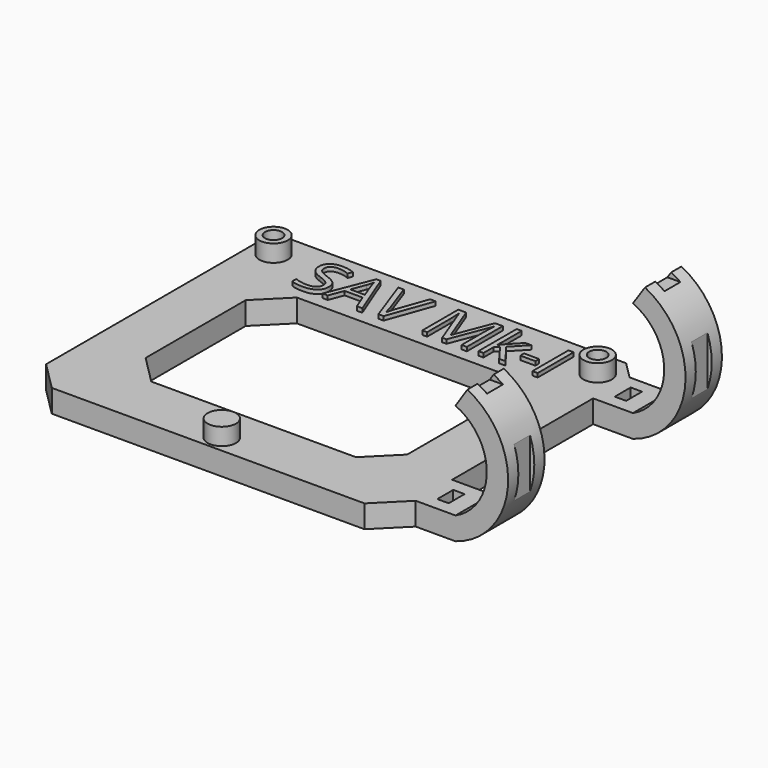
from build123d import *

# Parameters (mm, degrees)
F0_W          = 65
F0_H          = 55
F1_DEPTH      = 4
F2_W          = 46
F2_H          = 32
F3_DEPTH      = 4
F4_SIZE       = 5
F5_R          = 2.5
F6_DEPTH      = 3
F9_D          = 3
F9_ON_F8_D    = 3
F10_W         = 7
F10_H         = 8
F11_DEPTH     = 4
F12_SIZE      = 4.99999
F13_SIZE      = 2.99999
F14_SIZE      = 5
F15_SIZE      = 3
F16_TEXT_SIZE = 11.0753294494
F17_DEPTH     = 0.7
F19_DEPTH     = 8
F21_DEPTH     = 8
F22_W         = 7.0721879601
F22_H         = 3.5
F22_W_2       = 5.6506387591
F23_DEPTH     = 24.1616448952
F24_W         = 2
F24_H         = 3.5
F25_DEPTH     = 4.001
F26_W         = 3.5
F26_H         = 5.8661212551
F26_H_2       = 5.611290465
F27_DEPTH     = 81.2529563753


# Not quite as in the source:
# - a fillet or chamfer is up to 0.001 mm smaller than in the source, because OpenCascade refuses the exact size
# - Text() gives the source's letters only with a copy of the font that has no kerning and outlines rounded to 1/6400 em; it was checked with that copy


with BuildPart() as f1:
    # F0 (on Top) → F1 (new body)
    with BuildSketch(Plane.XY):
        with Locations((32.5, 27.5)):
            Rectangle(F0_W, F0_H)
    extrude(amount=F1_DEPTH)

    # F2 (on face) → F3 (cut, through all)
    with BuildSketch(Plane.XY.offset(4)):
        with Locations((32.5, 26)):
            Rectangle(F2_W, F2_H)
    extrude(amount=-F3_DEPTH, mode=Mode.SUBTRACT)

    # F4
    f4_edges = [f1.edges().sort_by_distance(p)[0] for p in [
        (9.5, 42, 2),
        (55.5, 42, 2),
        (9.5, 10, 2),
        (55.5, 10, 2),
    ]]
    chamfer(f4_edges, length=F4_SIZE)

    # F5 (on face) → F6 (join)
    with BuildSketch(Plane.XY.offset(4)):
        with Locations((32.5, 3)):
            Circle(F5_R)
        with Locations((4, 50)):
            Circle(F5_R)
        with Locations((61, 50)):
            Circle(F5_R)
    extrude(amount=F6_DEPTH)

    # F9 (through all)
    with Locations(Plane.XY.offset(7)):
        with Locations((4, 50)):
            Hole(F9_D / 2)

    # F9 on F8 (through all)
    with Locations(Plane.XY.offset(7)):
        with Locations((61, 50)):
            Hole(F9_ON_F8_D / 2)

    # F10 (on face) → F11 (join)
    with BuildSketch(Plane.XY.offset(4)):
        with Locations((68.5, 48)):
            Rectangle(F10_W, F10_H)
        with Locations((68.5, 9)):
            Rectangle(F10_W, F10_H)
    extrude(amount=-F11_DEPTH)

    # F12 (size 5 in the source; OpenCascade refuses exactly that, so slightly less here)
    f12_edges = [f1.edges().sort_by_distance(p)[0] for p in [
        (65, 0, 2),
    ]]
    chamfer(f12_edges, length=F12_SIZE)

    # F13 (size 3 in the source; OpenCascade refuses exactly that, so slightly less here)
    f13_edges = [f1.edges().sort_by_distance(p)[0] for p in [
        (65, 55, 2),
    ]]
    chamfer(f13_edges, length=F13_SIZE)

    # F14
    f14_edges = [f1.edges().sort_by_distance(p)[0] for p in [
        (0, 0, 2),
    ]]
    chamfer(f14_edges, length=F14_SIZE)

    # F15
    f15_edges = [f1.edges().sort_by_distance(p)[0] for p in [
        (0, 55, 2),
    ]]
    chamfer(f15_edges, length=F15_SIZE)

    # F16 (on face) → F17 (join)
    with BuildSketch(Plane.XY.offset(4)):
        with Locations((11.2528149039, 44.0769940615)):
            Text('SAV Mk-I', F16_TEXT_SIZE, font='Open Sans', text_align=(TextAlign.LEFT, TextAlign.BOTTOM))
    extrude(amount=F17_DEPTH)

    # F18 (on face) → F19 (join)
    with BuildSketch(Plane.XZ.offset(-5)):
        with BuildLine():
            ThreePointArc((72, 21), (77.5, 12.5), (72, 4))
            Line((72, 4), (72, 0))
            ThreePointArc((72, 0), (81.2035179843, 11.3757906555), (74.0858738239, 24.1606448952))
            Line((74.0858738239, 24.1606448952), (72, 21))
        make_face()
    extrude(amount=-F19_DEPTH)

    # F20 (on face) → F21 (join)
    with BuildSketch(Plane.XZ.offset(-44)):
        with BuildLine():
            ThreePointArc((72, 21), (77.5, 12.5), (72, 4))
            Line((72, 4), (72, 0))
            ThreePointArc((72, 0), (81.2016221654, 11.3540433579), (74.1247920887, 24.1408579383))
            Line((74.1247920887, 24.1408579383), (72, 21))
        make_face()
    extrude(amount=-F21_DEPTH)

    # F22 (on Top) → F23 (cut, through all)
    with BuildSketch(Plane.XY):
        with Locations((84.0360939801, 9)):
            Rectangle(F22_W, F22_H)
        with Locations((83.3253193796, 48)):
            Rectangle(F22_W_2, F22_H)
    extrude(amount=F23_DEPTH, mode=Mode.SUBTRACT)

    # F24 (on face) → F25 (cut, through all)
    with BuildSketch(Plane.XY.offset(4)):
        with Locations((68, 9)):
            Rectangle(F24_W, F24_H)
        with Locations((68, 48)):
            Rectangle(F24_W, F24_H)
    extrude(amount=-F25_DEPTH, mode=Mode.SUBTRACT)

    # F26 (on Right) → F27 (cut, through all)
    with BuildSketch(Plane.YZ):
        with Locations((9, 26.0937055228)):
            Rectangle(F26_W, F26_H)
        with Locations((48, 25.9662901277)):
            Rectangle(F26_W, F26_H_2)
    extrude(amount=F27_DEPTH, mode=Mode.SUBTRACT)


solid = f1.part
